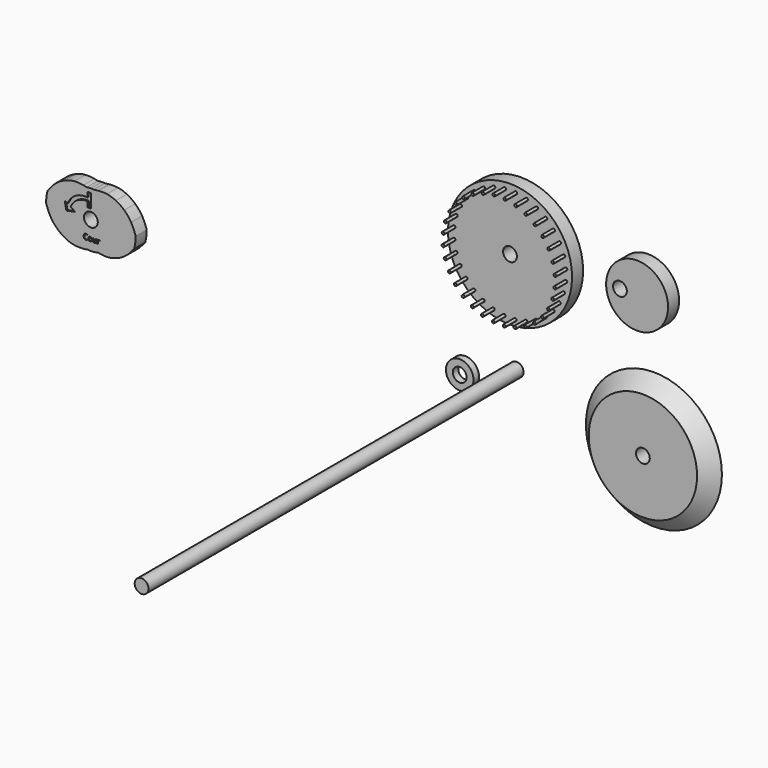
from build123d import *

# Parameters (mm, degrees)
F0_R          = 45
F1_DEPTH      = 10
F0_R_2        = 22.45
F0_R_3        = 49.315
F2_R          = 5
F3_DEPTH      = 10.0010001
F4_R          = 5
F5_DEPTH      = 10.0010001
F6_R          = 5
F7_DEPTH      = 10.0010001
F8_SIZE       = 9.99999
F9_R          = 5
F10_DEPTH     = 340
F11_R         = 10
F12_DEPTH     = 5
F13_R         = 5
F14_DEPTH     = 5.0010001
F16_DEPTH     = 10
F17_R         = 5
F18_DEPTH     = 25
F19_TEXT_SIZE = 5.3993426263
F20_DEPTH     = 1


# Not quite as in the source:
# - a fillet or chamfer is up to 0.001 mm smaller than in the source, because OpenCascade refuses the exact size
# - Text() gives the source's letters only with a copy of the font that has no kerning and outlines rounded to 1/6400 em; it was checked with that copy


with BuildPart() as f1:
    # F0 (on Front) → F1 (new body)
    with BuildSketch(Plane.XZ):
        with Locations((-46.6972251093, 45.5633398328)):
            Circle(F0_R)
    extrude(amount=F1_DEPTH)

    # F2 (on face) → F3 (cut, through all)
    with BuildSketch(Plane.XZ.offset(10)):
        with Locations((-46.6972251093, 45.5633398328)):
            Circle(F2_R)
    extrude(amount=-F3_DEPTH, mode=Mode.SUBTRACT)

    # F15 (on face) → F16 (join)
    with BuildSketch(Plane.XZ.offset(10)):
        with BuildLine():
            Line((-20.3267769857, 14.6089610016), (-21.0381806281, 13.9061773524))
            Line((-21.0381806281, 13.9061773524), (-21.8730211374, 13.3556854596))
            ThreePointArc((-21.8730211374, 13.3556854596), (-20.7508137105, 12.948356777), (-20.0381806281, 13.9061773524))
            ThreePointArc((-20.0381806281, 13.9061773524), (-20.1131391041, 14.2860433535), (-20.3267769857, 14.6089610016))
        make_face()
        with BuildLine():
            Line((-21.8730211374, 13.3556854596), (-21.0381806281, 13.9061773524))
            Line((-21.0381806281, 13.9061773524), (-20.3267769857, 14.6089610016))
            ThreePointArc((-20.3267769857, 14.6089610016), (-21.6678504313, 14.6830402353), (-21.8730211374, 13.3556854596))
        make_face()
        with BuildLine():
            ThreePointArc((-41.4559151977, 86.0920184473), (-42.4528675557, 87.0920138032), (-43.4558966214, 86.0981137029))
            Line((-43.4558966214, 86.0981137029), (-42.4559151977, 86.0920184473))
            Line((-42.4559151977, 86.0920184473), (-41.4763372619, 85.8909536123))
            ThreePointArc((-41.4763372619, 85.8909536123), (-41.4610338138, 85.9909687954), (-41.4559151977, 86.0920184473))
        make_face()
        with BuildLine():
            Line((-42.4559151977, 86.0920184473), (-43.4558966214, 86.0981137029))
            ThreePointArc((-43.4558966214, 86.0981137029), (-42.5599964225, 85.0974496469), (-41.4763372619, 85.8909536123))
            Line((-41.4763372619, 85.8909536123), (-42.4559151977, 86.0920184473))
        make_face()
        with BuildLine():
            ThreePointArc((-49.4441637401, 86.1407097685), (-50.5391474585, 87.1361885946), (-51.4261199266, 85.9516012075))
            Line((-51.4261199266, 85.9516012075), (-50.4441637401, 86.1407097685))
            Line((-50.4441637401, 86.1407097685), (-49.4441823163, 86.1346145129))
            ThreePointArc((-49.4441823163, 86.1346145129), (-49.4441683842, 86.1376621265), (-49.4441637401, 86.1407097685))
        make_face()
        with BuildLine():
            Line((-50.4441637401, 86.1407097685), (-51.4261199266, 85.9516012075))
            ThreePointArc((-51.4261199266, 85.9516012075), (-50.3522143259, 85.1449460891), (-49.4441823163, 86.1346145129))
            Line((-49.4441823163, 86.1346145129), (-50.4441637401, 86.1407097685))
        make_face()
        with BuildLine():
            ThreePointArc((-57.3064633458, 84.8191440801), (-58.5728660212, 85.5887274378), (-59.2146144559, 84.2529904775))
            Line((-59.2146144559, 84.2529904775), (-58.2884195323, 84.6300355191))
            Line((-58.2884195323, 84.6300355191), (-57.3064633458, 84.8191440801))
        make_face()
        with BuildLine():
            Line((-58.2884195323, 84.6300355191), (-59.2146144559, 84.2529904775))
            ThreePointArc((-59.2146144559, 84.2529904775), (-58.0963191987, 83.6486602281), (-57.2884195323, 84.6300355191))
            ThreePointArc((-57.2884195323, 84.6300355191), (-57.2929407062, 84.7250192375), (-57.3064633458, 84.8191440801))
            Line((-57.3064633458, 84.8191440801), (-58.2884195323, 84.6300355191))
        make_face()
        with BuildLine():
            ThreePointArc((-64.7610372996, 81.9950951051), (-66.1532446677, 82.5028282286), (-66.5220727325, 81.0675581706))
            Line((-66.5220727325, 81.0675581706), (-65.6872322232, 81.6180500634))
            Line((-65.6872322232, 81.6180500634), (-64.7610372996, 81.9950951051))
        make_face()
        with BuildLine():
            Line((-65.6872322232, 81.6180500634), (-66.5220727325, 81.0675581706))
            ThreePointArc((-66.5220727325, 81.0675581706), (-65.3998653056, 80.660229488), (-64.6872322232, 81.6180500634))
            ThreePointArc((-64.6872322232, 81.6180500634), (-64.7058569322, 81.810150397), (-64.7610372996, 81.9950951051))
            Line((-64.7610372996, 81.9950951051), (-65.6872322232, 81.6180500634))
        make_face()
        with BuildLine():
            ThreePointArc((-71.5214290812, 77.770994206), (-72.9859393937, 77.9973651962), (-73.0676732328, 76.517718664))
            Line((-73.0676732328, 76.517718664), (-72.3562695905, 77.2205023132))
            Line((-72.3562695905, 77.2205023132), (-71.5214290812, 77.770994206))
        make_face()
        with BuildLine():
            Line((-72.3562695905, 77.2205023132), (-73.0676732328, 76.517718664))
            ThreePointArc((-73.0676732328, 76.517718664), (-71.9764035893, 76.2954607892), (-71.3562695905, 77.2205023132))
            ThreePointArc((-71.3562695905, 77.2205023132), (-71.3984490151, 77.5078692309), (-71.5214290812, 77.770994206))
            Line((-71.5214290812, 77.770994206), (-72.3562695905, 77.2205023132))
        make_face()
        with BuildLine():
            ThreePointArc((-77.3278406257, 72.3091712117), (-78.8083735726, 72.2454807583), (-78.5998722005, 70.7783197384))
            Line((-78.5998722005, 70.7783197384), (-78.0392442681, 71.6063875625))
            Line((-78.0392442681, 71.6063875625), (-77.3278406257, 72.3091712117))
        make_face()
        with BuildLine():
            Line((-78.0392442681, 71.6063875625), (-78.5998722005, 70.7783197384))
            ThreePointArc((-78.5998722005, 70.7783197384), (-77.5705375007, 70.7230337454), (-77.0392442681, 71.6063875625))
            ThreePointArc((-77.0392442681, 71.6063875625), (-77.114202744, 71.9862535636), (-77.3278406257, 72.3091712117))
            Line((-77.3278406257, 72.3091712117), (-78.0392442681, 71.6063875625))
        make_face()
        with BuildLine():
            ThreePointArc((-81.9571347938, 65.8195209167), (-83.3967943242, 65.4682166082), (-82.9060703316, 64.0699232756))
            Line((-82.9060703316, 64.0699232756), (-82.5177627262, 64.9914530926))
            Line((-82.5177627262, 64.9914530926), (-81.9571347938, 65.8195209167))
        make_face()
        with BuildLine():
            Line((-82.5177627262, 64.9914530926), (-82.9060703316, 64.0699232756))
            ThreePointArc((-82.9060703316, 64.0699232756), (-81.964729095, 64.1582941626), (-81.5177627262, 64.9914530926))
            ThreePointArc((-81.5177627262, 64.9914530926), (-81.6344089091, 65.46015986), (-81.9571347938, 65.8195209167))
            Line((-81.9571347938, 65.8195209167), (-82.5177627262, 64.9914530926))
        make_face()
        with BuildLine():
            ThreePointArc((-85.2314104067, 58.5514369425), (-86.5748712122, 57.9260192064), (-85.820782847, 56.6503291898))
            Line((-85.820782847, 56.6503291898), (-85.6197180121, 57.6299071255))
            Line((-85.6197180121, 57.6299071255), (-85.2314104067, 58.5514369425))
        make_face()
        with BuildLine():
            Line((-85.6197180121, 57.6299071255), (-85.820782847, 56.6503291898))
            ThreePointArc((-85.820782847, 56.6503291898), (-84.9876835332, 56.8549668585), (-84.6197180121, 57.6299071255))
            ThreePointArc((-84.6197180121, 57.6299071255), (-84.786559082, 58.1829407568), (-85.2314104067, 58.5514369425))
            Line((-85.2314104067, 58.5514369425), (-85.6197180121, 57.6299071255))
        make_face()
        with BuildLine():
            ThreePointArc((-87.0248388888, 50.7842276802), (-88.2204725241, 49.9087309693), (-87.2319989793, 48.8046683207))
            Line((-87.2319989793, 48.8046683207), (-87.2259037237, 49.8046497444))
            Line((-87.2259037237, 49.8046497444), (-87.0248388888, 50.7842276802))
        make_face()
        with BuildLine():
            Line((-87.2259037237, 49.8046497444), (-87.2319989793, 48.8046683207))
            ThreePointArc((-87.2319989793, 48.8046683207), (-86.5209552347, 49.0953912388), (-86.2259037237, 49.8046497444))
            ThreePointArc((-86.2259037237, 49.8046497444), (-86.4509634567, 50.4366842233), (-87.0248388888, 50.7842276802))
            Line((-87.0248388888, 50.7842276802), (-87.2259037237, 49.8046497444))
        make_face()
        with BuildLine():
            ThreePointArc((-87.2684997893, 42.8163826257), (-88.2703587244, 41.7244517877), (-87.085486484, 40.8344450155))
            Line((-87.085486484, 40.8344450155), (-87.274595045, 41.816401202))
            Line((-87.274595045, 41.816401202), (-87.2684997893, 42.8163826257))
        make_face()
        with BuildLine():
            Line((-87.274595045, 41.816401202), (-87.085486484, 40.8344450155))
            ThreePointArc((-87.085486484, 40.8344450155), (-86.5035215851, 41.1796550049), (-86.274595045, 41.816401202))
            ThreePointArc((-86.274595045, 41.816401202), (-86.5653365393, 42.521349691), (-87.2684997893, 42.8163826257))
            Line((-87.2684997893, 42.8163826257), (-87.274595045, 41.816401202))
        make_face()
        with BuildLine():
            ThreePointArc((-85.9530293566, 34.9541015963), (-86.7226127143, 33.6876989209), (-85.386875754, 33.0459504862))
            Line((-85.386875754, 33.0459504862), (-85.7639207956, 33.9721454098))
            Line((-85.7639207956, 33.9721454098), (-85.9530293566, 34.9541015963))
        make_face()
        with BuildLine():
            Line((-85.7639207956, 33.9721454098), (-85.386875754, 33.0459504862))
            ThreePointArc((-85.386875754, 33.0459504862), (-84.9341482239, 33.4140437352), (-84.7639207956, 33.9721454098))
            ThreePointArc((-84.7639207956, 33.9721454098), (-85.1271745985, 34.7432188697), (-85.9530293566, 34.9541015963))
            Line((-85.9530293566, 34.9541015963), (-85.7639207956, 33.9721454098))
        make_face()
        with BuildLine():
            ThreePointArc((-83.1289803815, 27.4995276425), (-83.6367135051, 26.1073202744), (-82.2014434471, 25.7384922096))
            Line((-82.2014434471, 25.7384922096), (-82.7519353399, 26.5733327189))
            Line((-82.7519353399, 26.5733327189), (-83.1289803815, 27.4995276425))
        make_face()
        with BuildLine():
            Line((-82.7519353399, 26.5733327189), (-82.2014434471, 25.7384922096))
            ThreePointArc((-82.2014434471, 25.7384922096), (-81.8714548197, 26.099250391), (-81.7519353399, 26.5733327189))
            ThreePointArc((-81.7519353399, 26.5733327189), (-82.1938336653, 27.4031052906), (-83.1289803815, 27.4995276425))
            Line((-83.1289803815, 27.4995276425), (-82.7519353399, 26.5733327189))
        make_face()
        with BuildLine():
            ThreePointArc((-78.9048794825, 20.7391358609), (-79.1312504727, 19.2746255484), (-77.6516039405, 19.1928917093))
            Line((-77.6516039405, 19.1928917093), (-78.3543875897, 19.9042953516))
            Line((-78.3543875897, 19.9042953516), (-78.9048794825, 20.7391358609))
        make_face()
        with BuildLine():
            Line((-78.3543875897, 19.9042953516), (-77.6516039405, 19.1928917093))
            ThreePointArc((-77.6516039405, 19.1928917093), (-77.4316786299, 19.5187980424), (-77.3543875897, 19.9042953516))
            ThreePointArc((-77.3543875897, 19.9042953516), (-77.8803052618, 20.7847758718), (-78.9048794825, 20.7391358609))
            Line((-78.9048794825, 20.7391358609), (-78.3543875897, 19.9042953516))
        make_face()
        with BuildLine():
            ThreePointArc((-73.4430564882, 14.9327243164), (-73.3793660348, 13.4521913695), (-71.9122050148, 13.6606927416))
            Line((-71.9122050148, 13.6606927416), (-72.740272839, 14.221320674))
            Line((-72.740272839, 14.221320674), (-73.4430564882, 14.9327243164))
        make_face()
        with BuildLine():
            Line((-72.740272839, 14.221320674), (-71.9122050148, 13.6606927416))
            ThreePointArc((-71.9122050148, 13.6606927416), (-71.7842216311, 13.9281209334), (-71.740272839, 14.221320674))
            ThreePointArc((-71.740272839, 14.221320674), (-72.3547755298, 15.1440296339), (-73.4430564882, 14.9327243164))
            Line((-73.4430564882, 14.9327243164), (-72.740272839, 14.221320674))
        make_face()
        with BuildLine():
            ThreePointArc((-66.9534061932, 10.3034301483), (-66.6021018846, 8.8637706179), (-65.2038085521, 9.3544946105))
            Line((-65.2038085521, 9.3544946105), (-66.1253383691, 9.7428022159))
            Line((-66.1253383691, 9.7428022159), (-66.9534061932, 10.3034301483))
        make_face()
        with BuildLine():
            Line((-66.1253383691, 9.7428022159), (-65.2038085521, 9.3544946105))
            ThreePointArc((-65.2038085521, 9.3544946105), (-65.145152209, 9.5447237175), (-65.1253383691, 9.7428022159))
            ThreePointArc((-65.1253383691, 9.7428022159), (-65.8321386284, 10.6988534238), (-66.9534061932, 10.3034301483))
            Line((-66.9534061932, 10.3034301483), (-66.1253383691, 9.7428022159))
        make_face()
        with BuildLine():
            ThreePointArc((-59.685322219, 7.0291545354), (-59.0599044828, 5.6856937299), (-57.7842144663, 6.439782095))
            Line((-57.7842144663, 6.439782095), (-58.763792402, 6.64084693))
            Line((-58.763792402, 6.64084693), (-59.685322219, 7.0291545354))
        make_face()
        with BuildLine():
            Line((-58.763792402, 6.64084693), (-57.7842144663, 6.439782095))
            ThreePointArc((-57.7842144663, 6.439782095), (-57.7689110182, 6.5397972781), (-57.763792402, 6.64084693))
            ThreePointArc((-57.763792402, 6.64084693), (-58.5657139036, 7.6210330901), (-59.685322219, 7.0291545354))
            Line((-59.685322219, 7.0291545354), (-58.763792402, 6.64084693))
        make_face()
        with BuildLine():
            ThreePointArc((-51.9181129566, 5.2357260533), (-51.0426162457, 4.040092418), (-49.9385535972, 5.0285659628))
            Line((-49.9385535972, 5.0285659628), (-50.9385350209, 5.0346612184))
            Line((-50.9385350209, 5.0346612184), (-51.9181129566, 5.2357260533))
        make_face()
        with BuildLine():
            Line((-50.9385350209, 5.0346612184), (-49.9385535972, 5.0285659628))
            ThreePointArc((-49.9385535972, 5.0285659628), (-49.938539665, 5.0316135764), (-49.9385350209, 5.0346612184))
            ThreePointArc((-49.9385350209, 5.0346612184), (-50.8374853691, 6.0295426022), (-51.9181129566, 5.2357260533))
            Line((-51.9181129566, 5.2357260533), (-50.9385350209, 5.0346612184))
        make_face()
        with BuildLine():
            ThreePointArc((-41.9502864785, 4.9859698971), (-41.9548076523, 5.0809536155), (-41.968330292, 5.1750784581))
            Line((-41.968330292, 5.1750784581), (-42.9502864785, 4.9859698971))
            Line((-42.9502864785, 4.9859698971), (-43.9502679022, 4.9920651527))
            ThreePointArc((-43.9502679022, 4.9920651527), (-42.9533341204, 3.9859745412), (-41.9502864785, 4.9859698971))
        make_face()
        with BuildLine():
            Line((-42.9502864785, 4.9859698971), (-41.968330292, 5.1750784581))
            ThreePointArc((-41.968330292, 5.1750784581), (-43.0422358927, 5.9817335765), (-43.9502679022, 4.9920651527))
            Line((-43.9502679022, 4.9920651527), (-42.9502864785, 4.9859698971))
        make_face()
        with BuildLine():
            ThreePointArc((-34.1060306863, 6.4966441465), (-34.1246553953, 6.6887444801), (-34.1798357626, 6.8736891881))
            Line((-34.1798357626, 6.8736891881), (-35.1060306863, 6.4966441465))
            Line((-35.1060306863, 6.4966441465), (-36.0879868727, 6.3075355855))
            ThreePointArc((-36.0879868727, 6.3075355855), (-35.0110469679, 5.5011653204), (-34.1060306863, 6.4966441465))
        make_face()
        with BuildLine():
            Line((-35.1060306863, 6.4966441465), (-34.1798357626, 6.8736891881))
            ThreePointArc((-34.1798357626, 6.8736891881), (-35.3904771752, 7.4553360652), (-36.0879868727, 6.3075355855))
            Line((-36.0879868727, 6.3075355855), (-35.1060306863, 6.4966441465))
        make_face()
        with BuildLine():
            ThreePointArc((-26.7072179953, 9.5086296022), (-26.74939742, 9.7959965198), (-26.8723774861, 10.059121495))
            Line((-26.8723774861, 10.059121495), (-27.7072179953, 9.5086296022))
            Line((-27.7072179953, 9.5086296022), (-28.633412919, 9.1315845606))
            ThreePointArc((-28.633412919, 9.1315845606), (-27.5151176617, 8.5272543112), (-26.7072179953, 9.5086296022))
        make_face()
        with BuildLine():
            Line((-27.7072179953, 9.5086296022), (-26.8723774861, 10.059121495))
            ThreePointArc((-26.8723774861, 10.059121495), (-28.1732304399, 10.3934077674), (-28.633412919, 9.1315845606))
            Line((-28.633412919, 9.1315845606), (-27.7072179953, 9.5086296022))
        make_face()
        with BuildLine():
            ThreePointArc((-35.6102357523, 84.6868975706), (-34.9267698973, 83.5306795356), (-33.7091279996, 84.0975251302))
            Line((-33.7091279996, 84.0975251302), (-34.6306578165, 84.4858327356))
            Line((-34.6306578165, 84.4858327356), (-35.6102357523, 84.6868975706))
        make_face()
        with BuildLine():
            Line((-34.6306578165, 84.4858327356), (-33.7091279996, 84.0975251302))
            ThreePointArc((-33.7091279996, 84.0975251302), (-33.6504716564, 84.2877542373), (-33.6306578165, 84.4858327356))
            ThreePointArc((-33.6306578165, 84.4858327356), (-34.5296081647, 85.4807141194), (-35.6102357523, 84.6868975706))
            Line((-35.6102357523, 84.6868975706), (-34.6306578165, 84.4858327356))
        make_face()
        with BuildLine():
            ThreePointArc((-28.1906416665, 81.7721850552), (-27.7458753651, 80.5048458518), (-26.4410440253, 80.8232495173))
            Line((-26.4410440253, 80.8232495173), (-27.2691118495, 81.3838774497))
            Line((-27.2691118495, 81.3838774497), (-28.1906416665, 81.7721850552))
        make_face()
        with BuildLine():
            Line((-27.2691118495, 81.3838774497), (-26.4410440253, 80.8232495173))
            ThreePointArc((-26.4410440253, 80.8232495173), (-26.3130606416, 81.0906777091), (-26.2691118495, 81.3838774497))
            ThreePointArc((-26.2691118495, 81.3838774497), (-27.0710333511, 82.3640636098), (-28.1906416665, 81.7721850552))
            Line((-28.1906416665, 81.7721850552), (-27.2691118495, 81.3838774497))
        make_face()
        with BuildLine():
            ThreePointArc((-21.4822452037, 77.465986924), (-21.2932705754, 76.1362296871), (-19.9513937304, 76.1939553492))
            Line((-19.9513937304, 76.1939553492), (-20.6541773796, 76.9053589916))
            Line((-20.6541773796, 76.9053589916), (-21.4822452037, 77.465986924))
        make_face()
        with BuildLine():
            Line((-20.6541773796, 76.9053589916), (-19.9513937304, 76.1939553492))
            ThreePointArc((-19.9513937304, 76.1939553492), (-19.7314684197, 76.5198616824), (-19.6541773796, 76.9053589916))
            ThreePointArc((-19.6541773796, 76.9053589916), (-20.3609776389, 77.8614101995), (-21.4822452037, 77.465986924))
            Line((-21.4822452037, 77.465986924), (-20.6541773796, 76.9053589916))
        make_face()
        with BuildLine():
            ThreePointArc((-15.7428462781, 71.9337879564), (-15.8169255118, 70.5927145108), (-14.489570736, 70.3875438047))
            Line((-14.489570736, 70.3875438047), (-15.0400626288, 71.222384314))
            Line((-15.0400626288, 71.222384314), (-15.7428462781, 71.9337879564))
        make_face()
        with BuildLine():
            Line((-15.0400626288, 71.222384314), (-14.489570736, 70.3875438047))
            ThreePointArc((-14.489570736, 70.3875438047), (-14.1595821087, 70.7483019861), (-14.0400626288, 71.222384314))
            ThreePointArc((-14.0400626288, 71.222384314), (-14.6545653197, 72.1450932739), (-15.7428462781, 71.9337879564))
            Line((-15.7428462781, 71.9337879564), (-15.0400626288, 71.222384314))
        make_face()
        with BuildLine():
            ThreePointArc((-11.1930067715, 65.388187456), (-11.5272930438, 64.0873345022), (-10.265469837, 63.6271520231))
            Line((-10.265469837, 63.6271520231), (-10.6425148787, 64.5533469467))
            Line((-10.6425148787, 64.5533469467), (-11.1930067715, 65.388187456))
        make_face()
        with BuildLine():
            Line((-10.6425148787, 64.5533469467), (-10.265469837, 63.6271520231))
            ThreePointArc((-10.265469837, 63.6271520231), (-9.8127423069, 63.9952452722), (-9.6425148787, 64.5533469467))
            ThreePointArc((-9.6425148787, 64.5533469467), (-10.1684325508, 65.4338274669), (-11.1930067715, 65.388187456))
            Line((-11.1930067715, 65.388187456), (-10.6425148787, 64.5533469467))
        make_face()
        with BuildLine():
            ThreePointArc((-8.0075744646, 58.0807291795), (-8.5892213416, 56.8700877669), (-7.441420862, 56.1725780693))
            Line((-7.441420862, 56.1725780693), (-7.630529423, 57.1545342558))
            Line((-7.630529423, 57.1545342558), (-8.0075744646, 58.0807291795))
        make_face()
        with BuildLine():
            Line((-7.630529423, 57.1545342558), (-7.441420862, 56.1725780693))
            ThreePointArc((-7.441420862, 56.1725780693), (-6.8594559631, 56.5177880587), (-6.630529423, 57.1545342558))
            ThreePointArc((-6.630529423, 57.1545342558), (-7.0724277484, 57.9843068276), (-8.0075744646, 58.0807291795))
            Line((-8.0075744646, 58.0807291795), (-7.630529423, 57.1545342558))
        make_face()
        with BuildLine():
            ThreePointArc((-6.3089637346, 50.2922346501), (-7.115618853, 49.2183290494), (-6.1259504292, 48.3102970399))
            Line((-6.1259504292, 48.3102970399), (-6.1198551736, 49.3102784636))
            Line((-6.1198551736, 49.3102784636), (-6.3089637346, 50.2922346501))
        make_face()
        with BuildLine():
            Line((-6.1198551736, 49.3102784636), (-6.1259504292, 48.3102970399))
            ThreePointArc((-6.1259504292, 48.3102970399), (-5.4149066846, 48.601019958), (-5.1198551736, 49.3102784636))
            ThreePointArc((-5.1198551736, 49.3102784636), (-5.4831089765, 50.0813519235), (-6.3089637346, 50.2922346501))
            Line((-6.3089637346, 50.2922346501), (-6.1198551736, 49.3102784636))
        make_face()
        with BuildLine():
            ThreePointArc((-6.1624512392, 42.3220113449), (-7.1631152952, 41.426111146), (-6.3696113298, 40.3424519855))
            Line((-6.3696113298, 40.3424519855), (-6.1685464948, 41.3220299212))
            Line((-6.1685464948, 41.3220299212), (-6.1624512392, 42.3220113449))
        make_face()
        with BuildLine():
            Line((-6.1685464948, 41.3220299212), (-6.3696113298, 40.3424519855))
            ThreePointArc((-6.3696113298, 40.3424519855), (-5.5365120159, 40.5470896541), (-5.1685464948, 41.3220299212))
            ThreePointArc((-5.1685464948, 41.3220299212), (-5.4592879892, 42.0269784102), (-6.1624512392, 42.3220113449))
            Line((-6.1624512392, 42.3220113449), (-6.1685464948, 41.3220299212))
        make_face()
        with BuildLine():
            ThreePointArc((-7.5736673715, 34.4763504758), (-8.7298854065, 33.7928846209), (-8.1630398119, 32.5752427231))
            Line((-8.1630398119, 32.5752427231), (-7.7747322065, 33.4967725401))
            Line((-7.7747322065, 33.4967725401), (-7.5736673715, 34.4763504758))
        make_face()
        with BuildLine():
            Line((-7.7747322065, 33.4967725401), (-8.1630398119, 32.5752427231))
            ThreePointArc((-8.1630398119, 32.5752427231), (-7.2216985752, 32.66361361), (-6.7747322065, 33.4967725401))
            ThreePointArc((-6.7747322065, 33.4967725401), (-6.9997919394, 34.128807019), (-7.5736673715, 34.4763504758))
            Line((-7.5736673715, 34.4763504758), (-7.7747322065, 33.4967725401))
        make_face()
        with BuildLine():
            ThreePointArc((-10.4883798869, 27.05675639), (-11.7557190903, 26.6119900886), (-11.4373154248, 25.3071587489))
            Line((-11.4373154248, 25.3071587489), (-10.8766874924, 26.135226573))
            Line((-10.8766874924, 26.135226573), (-10.4883798869, 27.05675639))
        make_face()
        with BuildLine():
            Line((-10.8766874924, 26.135226573), (-11.4373154248, 25.3071587489))
            ThreePointArc((-11.4373154248, 25.3071587489), (-10.407980725, 25.2518727559), (-9.8766874924, 26.135226573))
            ThreePointArc((-9.8766874924, 26.135226573), (-10.0435285623, 26.6882602043), (-10.4883798869, 27.05675639))
            Line((-10.4883798869, 27.05675639), (-10.8766874924, 26.135226573))
        make_face()
        with BuildLine():
            ThreePointArc((-14.7945780181, 20.3483599273), (-16.124335255, 20.1593852989), (-16.0666095929, 18.8175084539))
            Line((-16.0666095929, 18.8175084539), (-15.3552059505, 19.5202921031))
            Line((-15.3552059505, 19.5202921031), (-14.7945780181, 20.3483599273))
        make_face()
        with BuildLine():
            Line((-15.3552059505, 19.5202921031), (-16.0666095929, 18.8175084539))
            ThreePointArc((-16.0666095929, 18.8175084539), (-14.9753399494, 18.5952505791), (-14.3552059505, 19.5202921031))
            ThreePointArc((-14.3552059505, 19.5202921031), (-14.4718521334, 19.9889988705), (-14.7945780181, 20.3483599273))
            Line((-14.7945780181, 20.3483599273), (-15.3552059505, 19.5202921031))
        make_face()
    extrude(amount=F16_DEPTH)


with BuildPart() as f1b:
    # F0 (on Front) → F1, piece 2 (new body)
    with BuildSketch(Plane.XZ):
        with Locations((45.457674756, 49.0673256573)):
            Circle(F0_R_2)
    extrude(amount=F1_DEPTH)

    # F6 (on face) → F7 (cut, through all)
    with BuildSketch(Plane.XZ.offset(10)):
        with Locations((33.0115074419, 49.3762256208)):
            Circle(F6_R)
    extrude(amount=-F7_DEPTH, mode=Mode.SUBTRACT)


with BuildPart() as f1c:
    # F0 (on Front) → F1, piece 3 (new body)
    with BuildSketch(Plane.XZ):
        with Locations((49.6624586107, -51.8475387692)):
            Circle(F0_R_3)
    extrude(amount=F1_DEPTH)

    # F4 (on face) → F5 (cut, through all)
    with BuildSketch(Plane.XZ.offset(10)):
        with Locations((49.6624586107, -51.8475387692)):
            Circle(F4_R)
    extrude(amount=-F5_DEPTH, mode=Mode.SUBTRACT)

    # F8 (size 10 in the source; OpenCascade refuses exactly that, so slightly less here)
    f8_edges = [f1c.edges().sort_by_distance(p)[0] for p in [
        (0.347459, -10, -51.847539),
    ]]
    chamfer(f8_edges, length=F8_SIZE)


with BuildPart() as f1d:
    # F0 (on Front) → F1, piece 4 (new body)
    with BuildSketch(Plane.XZ):
        with BuildLine():
            ThreePointArc((-331.3206634485, -36.470353457), (-330.8102827468, -33.9044963994), (-330.6391799743, -31.293972555))
            ThreePointArc((-330.6391799743, -31.293972555), (-330.8102827468, -28.6834487106), (-331.3206634485, -26.1175916529))
            ThreePointArc((-331.3206634485, -26.1175916529), (-332.1615893241, -23.6403039077), (-333.3186718986, -21.293972555))
            ThreePointArc((-333.3186718986, -21.293972555), (-334.7721131685, -19.1187439748), (-336.4970443506, -17.1518369312))
            ThreePointArc((-336.4970443506, -17.1518369312), (-338.4639513941, -15.4269057491), (-340.6391799743, -13.9734644793))
            ThreePointArc((-340.6391799743, -13.9734644793), (-342.985511327, -12.8163819047), (-345.4627990723, -11.9754560292))
            ThreePointArc((-345.4627990723, -11.9754560292), (-347.037380693, -11.6209696846), (-348.6354187421, -11.3946021899))
            ThreePointArc((-348.6354187421, -11.3946021899), (-349.6360367394, -11.319145806), (-350.6391799743, -11.293972555))
            ThreePointArc((-350.6391799743, -11.293972555), (-352.1457160849, -11.3507945497), (-353.6436917567, -11.5209376602))
            ThreePointArc((-353.6436917567, -11.5209376602), (-354.7359345454, -11.7180536242), (-355.8155608764, -11.9754560292))
            ThreePointArc((-355.8155608764, -11.9754560292), (-358.2928486216, -12.8163819047), (-360.6391799743, -13.9734644793))
            ThreePointArc((-360.6391799743, -13.9734644793), (-362.8144085545, -15.4269057491), (-364.781315598, -17.1518369312))
            ThreePointArc((-364.781315598, -17.1518369312), (-366.5062467801, -19.1187439748), (-367.95968805, -21.293972555))
            ThreePointArc((-367.95968805, -21.293972555), (-369.1167706245, -23.6403039077), (-369.9576965001, -26.1175916529))
            ThreePointArc((-369.9576965001, -26.1175916529), (-370.4680772018, -28.6834487106), (-370.6391799743, -31.293972555))
            ThreePointArc((-370.6391799743, -31.293972555), (-370.4680772018, -33.9044963994), (-369.9576965001, -36.470353457))
            ThreePointArc((-369.9576965001, -36.470353457), (-369.1167706245, -38.9476412023), (-367.95968805, -41.293972555))
            ThreePointArc((-367.95968805, -41.293972555), (-366.5062467801, -43.4692011351), (-364.781315598, -45.4361081787))
            ThreePointArc((-364.781315598, -45.4361081787), (-362.8144085545, -47.1610393608), (-360.6391799743, -48.6144806306))
            ThreePointArc((-360.6391799743, -48.6144806306), (-358.2928486216, -49.7715632052), (-355.8155608764, -50.6124890807))
            ThreePointArc((-355.8155608764, -50.6124890807), (-354.2394341305, -50.9672582493), (-352.6398153961, -51.1936574246))
            ThreePointArc((-352.6398153961, -51.1936574246), (-351.6407543869, -51.268878029), (-350.6391799743, -51.293972555))
            ThreePointArc((-350.6391799743, -51.293972555), (-348.0286561299, -51.1228697824), (-345.4627990723, -50.6124890807))
            ThreePointArc((-345.4627990723, -50.6124890807), (-342.985511327, -49.7715632052), (-340.6391799743, -48.6144806306))
            ThreePointArc((-340.6391799743, -48.6144806306), (-338.4639513941, -47.1610393608), (-336.4970443506, -45.4361081787))
            ThreePointArc((-336.4970443506, -45.4361081787), (-334.7721131685, -43.4692011351), (-333.3186718986, -41.293972555))
            ThreePointArc((-333.3186718986, -41.293972555), (-332.1615893241, -38.9476412023), (-331.3206634485, -36.470353457))
        make_face()
        with BuildLine():
            Line((-318.1391799743, -31.293972555), (-330.6391799743, -31.293972555))
            ThreePointArc((-330.6391799743, -31.293972555), (-330.8102827468, -33.9044963994), (-331.3206634485, -36.470353457))
            Line((-331.3206634485, -36.470353457), (-319.2465906199, -39.7055915208))
            ThreePointArc((-319.2465906199, -39.7055915208), (-318.4172219797, -35.5360738021), (-318.1391799743, -31.293972555))
        make_face()
        with BuildLine():
            ThreePointArc((-331.3206634485, -26.1175916529), (-330.8102827468, -28.6834487106), (-330.6391799743, -31.293972555))
            Line((-330.6391799743, -31.293972555), (-318.1391799743, -31.293972555))
            add(Edge.make_bspline(
                [(-321.4682200204, -23.4776373929), (-320.0791480854, -25.8891723509), (-319.1091640299, -28.5915724529), (-318.1391799743, -31.293972555)],
                knots=[0.8106564665, 0.8106564665, 0.8106564665, 0.8106564665, 1, 1, 1, 1], degree=3))
            Line((-321.4682200204, -23.4776373929), (-331.3206634485, -26.1175916529))
        make_face()
        with BuildLine():
            ThreePointArc((-333.3186718986, -21.293972555), (-332.1615893241, -23.6403039077), (-331.3206634485, -26.1175916529))
            Line((-331.3206634485, -26.1175916529), (-321.4682200204, -23.4776373929))
            add(Edge.make_bspline(
                [(-326.4770712087, -17.343972555), (-324.5410444938, -19.0922749893), (-322.8093135762, -21.149396565), (-321.4682200204, -23.4776373929)],
                knots=[0.627852836, 0.627852836, 0.627852836, 0.627852836, 0.8106564665, 0.8106564665, 0.8106564665, 0.8106564665], degree=3))
            Line((-326.4770712087, -17.343972555), (-333.3186718986, -21.293972555))
        make_face()
        with BuildLine():
            Line((-319.2465906199, -39.7055915208), (-331.3206634485, -36.470353457))
            ThreePointArc((-331.3206634485, -36.470353457), (-332.1615893241, -38.9476412023), (-333.3186718986, -41.293972555))
            Line((-333.3186718986, -41.293972555), (-325.2040138652, -45.978972555))
            add(Edge.make_bspline(
                [(-319.2465906199, -39.7055915208), (-321.1336024153, -41.9533240414), (-323.0206142106, -44.201056562), (-325.2040138652, -45.978972555)],
                knots=[0, 0, 0, 0, 0.2683906872, 0.2683906872, 0.2683906872, 0.2683906872], degree=3))
        make_face()
        with BuildLine():
            ThreePointArc((-336.4970443506, -17.1518369312), (-334.7721131685, -19.1187439748), (-333.3186718986, -21.293972555))
            Line((-333.3186718986, -21.293972555), (-326.4770712087, -17.343972555))
            add(Edge.make_bspline(
                [(-332.5372463759, -13.1920389566), (-330.395934388, -14.2627108581), (-328.3417454917, -15.6601039579), (-326.4770712087, -17.343972555)],
                knots=[0.4517864492, 0.4517864492, 0.4517864492, 0.4517864492, 0.627852836, 0.627852836, 0.627852836, 0.627852836], degree=3))
            Line((-332.5372463759, -13.1920389566), (-336.4970443506, -17.1518369312))
        make_face()
        with BuildLine():
            Line((-325.2040138652, -45.978972555), (-333.3186718986, -41.293972555))
            ThreePointArc((-333.3186718986, -41.293972555), (-334.7721131685, -43.4692011351), (-336.4970443506, -45.4361081787))
            Line((-336.4970443506, -45.4361081787), (-332.0776269682, -49.8555255611))
            add(Edge.make_bspline(
                [(-325.2040138652, -45.978972555), (-327.2893106377, -47.6770045548), (-329.6449594667, -48.9464904436), (-332.0776269682, -49.8555255611)],
                knots=[0.2683906872, 0.2683906872, 0.2683906872, 0.2683906872, 0.5247222446, 0.5247222446, 0.5247222446, 0.5247222446], degree=3))
        make_face()
        with BuildLine():
            ThreePointArc((-340.6391799743, -13.9734644793), (-338.4639513941, -15.4269057491), (-336.4970443506, -17.1518369312))
            Line((-336.4970443506, -17.1518369312), (-332.5372463759, -13.1920389566))
            add(Edge.make_bspline(
                [(-338.9891799743, -11.1155806468), (-336.7312968284, -11.436625491), (-334.5940794305, -12.1636071493), (-332.5372463759, -13.1920389566)],
                knots=[0.2826662246, 0.2826662246, 0.2826662246, 0.2826662246, 0.4517864492, 0.4517864492, 0.4517864492, 0.4517864492], degree=3))
            Line((-338.9891799743, -11.1155806468), (-340.6391799743, -13.9734644793))
        make_face()
        with BuildLine():
            Line((-332.0776269682, -49.8555255611), (-336.4970443506, -45.4361081787))
            ThreePointArc((-336.4970443506, -45.4361081787), (-338.4639513941, -47.1610393608), (-340.6391799743, -48.6144806306))
            Line((-340.6391799743, -48.6144806306), (-339.0791799743, -51.3164798905))
            add(Edge.make_bspline(
                [(-332.0776269682, -49.8555255611), (-334.3935818988, -50.7209477206), (-336.7793425041, -51.2596762552), (-339.0791799743, -51.3164798905)],
                knots=[0.5247222446, 0.5247222446, 0.5247222446, 0.5247222446, 0.768755732, 0.768755732, 0.768755732, 0.768755732], degree=3))
        make_face()
        with BuildLine():
            ThreePointArc((-345.4627990723, -11.9754560292), (-342.985511327, -12.8163819047), (-340.6391799743, -13.9734644793))
            Line((-340.6391799743, -13.9734644793), (-338.9891799743, -11.1155806468))
            add(Edge.make_bspline(
                [(-345.2039800272, -11.0095302029), (-343.4242888791, -10.8729632986), (-341.1514054001, -10.808137223), (-338.9891799743, -11.1155806468)],
                knots=[0.1207109657, 0.1207109657, 0.1207109657, 0.1207109657, 0.2826662246, 0.2826662246, 0.2826662246, 0.2826662246], degree=3))
            Line((-345.2039800272, -11.0095302029), (-345.4627990723, -11.9754560292))
        make_face()
        with BuildLine():
            Line((-339.0791799743, -51.3164798905), (-340.6391799743, -48.6144806306))
            ThreePointArc((-340.6391799743, -48.6144806306), (-342.985511327, -49.7715632052), (-345.4627990723, -50.6124890807))
            add(Edge.make_bspline(
                [(-339.0791799743, -51.3164798905), (-341.2584883873, -51.3703065812), (-343.3606437298, -50.991397831), (-345.4627990723, -50.6124890807)],
                knots=[0.768755732, 0.768755732, 0.768755732, 0.768755732, 1, 1, 1, 1], degree=3))
        make_face()
        with BuildLine():
            ThreePointArc((-348.6354187421, -11.3946021899), (-347.037380693, -11.6209696846), (-345.4627990723, -11.9754560292))
            Line((-345.4627990723, -11.9754560292), (-345.2039800272, -11.0095302029))
            add(Edge.make_bspline(
                [(-348.6354187421, -11.3946021899), (-347.5829326704, -11.2529602612), (-346.5304465987, -11.1113183325), (-345.2039800272, -11.0095302029)],
                knots=[0, 0, 0, 0, 0.1207109657, 0.1207109657, 0.1207109657, 0.1207109657], degree=3))
        make_face()
        with BuildLine():
            add(Edge.make_bspline(
                [(-352.6398153961, -51.1936574246), (-353.6934040957, -51.3351662186), (-354.7469927953, -51.4766750126), (-356.0743799215, -51.578414907)],
                knots=[0, 0, 0, 0, 0.1207581565, 0.1207581565, 0.1207581565, 0.1207581565], degree=3))
            ThreePointArc((-352.6398153961, -51.1936574246), (-354.2394341305, -50.9672582493), (-355.8155608764, -50.6124890807))
            Line((-355.8155608764, -50.6124890807), (-356.0743799215, -51.578414907))
        make_face()
        with BuildLine():
            ThreePointArc((-355.8155608764, -11.9754560292), (-354.7359345454, -11.7180536242), (-353.6436917567, -11.5209376602))
            add(Edge.make_bspline(
                [(-356.0743799215, -11.0095302029), (-355.0493997027, -11.1789532798), (-354.3465457297, -11.34994547), (-353.6436917567, -11.5209376602)],
                knots=[0.8744321336, 0.8744321336, 0.8744321336, 0.8744321336, 1, 1, 1, 1], degree=3))
            Line((-356.0743799215, -11.0095302029), (-355.8155608764, -11.9754560292))
        make_face()
        with BuildLine():
            Line((-356.0743799215, -51.578414907), (-355.8155608764, -50.6124890807))
            ThreePointArc((-355.8155608764, -50.6124890807), (-358.2928486216, -49.7715632052), (-360.6391799743, -48.6144806306))
            Line((-360.6391799743, -48.6144806306), (-362.2891799743, -51.4723644631))
            add(Edge.make_bspline(
                [(-356.0743799215, -51.578414907), (-357.8545146496, -51.7148564287), (-360.1270759624, -51.779773568), (-362.2891799743, -51.4723644631)],
                knots=[0.1207581565, 0.1207581565, 0.1207581565, 0.1207581565, 0.2827047234, 0.2827047234, 0.2827047234, 0.2827047234], degree=3))
        make_face()
        with BuildLine():
            ThreePointArc((-360.6391799743, -13.9734644793), (-358.2928486216, -12.8163819047), (-355.8155608764, -11.9754560292))
            Line((-355.8155608764, -11.9754560292), (-356.0743799215, -11.0095302029))
            add(Edge.make_bspline(
                [(-362.5741799743, -10.6219461666), (-360.2378534811, -10.4650249719), (-357.7339033751, -10.7352209386), (-356.0743799215, -11.0095302029)],
                knots=[0.6711278985, 0.6711278985, 0.6711278985, 0.6711278985, 0.8744321336, 0.8744321336, 0.8744321336, 0.8744321336], degree=3))
            Line((-362.5741799743, -10.6219461666), (-360.6391799743, -13.9734644793))
        make_face()
        with BuildLine():
            Line((-362.2891799743, -51.4723644631), (-360.6391799743, -48.6144806306))
            ThreePointArc((-360.6391799743, -48.6144806306), (-362.8144085545, -47.1610393608), (-364.781315598, -45.4361081787))
            Line((-364.781315598, -45.4361081787), (-368.7411135727, -49.3959061533))
            add(Edge.make_bspline(
                [(-362.2891799743, -51.4723644631), (-364.546936335, -51.1513554561), (-366.6842458557, -50.4243477583), (-368.7411135727, -49.3959061533)],
                knots=[0.2827047234, 0.2827047234, 0.2827047234, 0.2827047234, 0.4518158714, 0.4518158714, 0.4518158714, 0.4518158714], degree=3))
        make_face()
        with BuildLine():
            ThreePointArc((-364.781315598, -17.1518369312), (-362.8144085545, -15.4269057491), (-360.6391799743, -13.9734644793))
            Line((-360.6391799743, -13.9734644793), (-362.5741799743, -10.6219461666))
            add(Edge.make_bspline(
                [(-369.5542863711, -12.3788661582), (-367.3016801571, -11.4240651537), (-365.0305779705, -10.7869320577), (-362.5741799743, -10.6219461666)],
                knots=[0.4573751901, 0.4573751901, 0.4573751901, 0.4573751901, 0.6711278985, 0.6711278985, 0.6711278985, 0.6711278985], degree=3))
            Line((-369.5542863711, -12.3788661582), (-364.781315598, -17.1518369312))
        make_face()
        with BuildLine():
            Line((-368.7411135727, -49.3959061533), (-364.781315598, -45.4361081787))
            ThreePointArc((-364.781315598, -45.4361081787), (-366.5062467801, -43.4692011351), (-367.95968805, -41.293972555))
            Line((-367.95968805, -41.293972555), (-374.8012887399, -45.243972555))
            add(Edge.make_bspline(
                [(-368.7411135727, -49.3959061533), (-370.8824616467, -48.3252240517), (-372.9366243517, -46.9278383551), (-374.8012887399, -45.243972555)],
                knots=[0.4518158714, 0.4518158714, 0.4518158714, 0.4518158714, 0.6278728089, 0.6278728089, 0.6278728089, 0.6278728089], degree=3))
        make_face()
        with BuildLine():
            ThreePointArc((-367.95968805, -21.293972555), (-366.5062467801, -19.1187439748), (-364.781315598, -17.1518369312))
            Line((-364.781315598, -17.1518369312), (-369.5542863711, -12.3788661582))
            add(Edge.make_bspline(
                [(-376.2908524344, -16.483972555), (-374.250519467, -14.7261911279), (-371.9125386988, -13.3784468561), (-369.5542863711, -12.3788661582)],
                knots=[0.2335975858, 0.2335975858, 0.2335975858, 0.2335975858, 0.4573751901, 0.4573751901, 0.4573751901, 0.4573751901], degree=3))
            Line((-376.2908524344, -16.483972555), (-367.95968805, -21.293972555))
        make_face()
        with BuildLine():
            Line((-374.8012887399, -45.243972555), (-367.95968805, -41.293972555))
            ThreePointArc((-367.95968805, -41.293972555), (-369.1167706245, -38.9476412023), (-369.9576965001, -36.470353457))
            Line((-369.9576965001, -36.470353457), (-379.8101399282, -39.1103077171))
            add(Edge.make_bspline(
                [(-374.8012887399, -45.243972555), (-376.7373051814, -43.4956730245), (-378.4690433931, -41.4385493871), (-379.8101399282, -39.1103077171)],
                knots=[0.6278728089, 0.6278728089, 0.6278728089, 0.6278728089, 0.8106666284, 0.8106666284, 0.8106666284, 0.8106666284], degree=3))
        make_face()
        with BuildLine():
            ThreePointArc((-369.9576965001, -26.1175916529), (-369.1167706245, -23.6403039077), (-367.95968805, -21.293972555))
            Line((-367.95968805, -21.293972555), (-376.2908524344, -16.483972555))
            add(Edge.make_bspline(
                [(-382.0317693287, -22.8823535891), (-380.2262450976, -20.6006219457), (-378.4207208666, -18.3188903022), (-376.2908524344, -16.483972555)],
                knots=[0, 0, 0, 0, 0.2335975858, 0.2335975858, 0.2335975858, 0.2335975858], degree=3))
            Line((-382.0317693287, -22.8823535891), (-369.9576965001, -26.1175916529))
        make_face()
        with BuildLine():
            Line((-379.8101399282, -39.1103077171), (-369.9576965001, -36.470353457))
            ThreePointArc((-369.9576965001, -36.470353457), (-370.4680772018, -33.9044963994), (-370.6391799743, -31.293972555))
            Line((-370.6391799743, -31.293972555), (-383.1391799743, -31.293972555))
            add(Edge.make_bspline(
                [(-379.8101399282, -39.1103077171), (-381.1992149492, -36.6987718867), (-382.1691974617, -33.9963722208), (-383.1391799743, -31.293972555)],
                knots=[0.8106666284, 0.8106666284, 0.8106666284, 0.8106666284, 1, 1, 1, 1], degree=3))
        make_face()
        with BuildLine():
            ThreePointArc((-370.6391799743, -31.293972555), (-370.4680772018, -28.6834487106), (-369.9576965001, -26.1175916529))
            Line((-369.9576965001, -26.1175916529), (-382.0317693287, -22.8823535891))
            ThreePointArc((-382.0317693287, -22.8823535891), (-382.861137969, -27.0518713078), (-383.1391799743, -31.293972555))
            Line((-383.1391799743, -31.293972555), (-370.6391799743, -31.293972555))
        make_face()
    extrude(amount=F1_DEPTH)

    # F17 (on face) → F18 (cut)
    with BuildSketch(Plane.XZ.offset(10)):
        with Locations((-350.6391799743, -31.293972555)):
            Circle(F17_R)
    extrude(amount=-F18_DEPTH, mode=Mode.SUBTRACT)

    # F19 (on face) → F20 (cut)
    with BuildSketch(Plane.XZ.offset(10)):
        with BuildLine():
            Line((-350.7084548473, -24.2036078125), (-350.7084548473, -14.2780067399))
            Line((-350.7084548473, -14.2780067399), (-353.0244231224, -14.2780067399))
            Line((-353.0244231224, -14.2780067399), (-353.0244231224, -17.9173927754))
            ThreePointArc((-353.0244231224, -17.9173927754), (-361.6815373497, -19.5773649411), (-367.4165606499, -26.2714400887))
            Line((-367.4165606499, -26.2714400887), (-369.649797678, -25.3615938127))
            Line((-369.649797678, -25.3615938127), (-368.4090971947, -31.3169546425))
            Line((-368.4090971947, -31.3169546425), (-361.945074023, -29.9702828115))
            Line((-361.945074023, -29.9702828115), (-365.348726511, -28.0084200203))
            ThreePointArc((-365.348726511, -28.0084200203), (-360.4589782524, -22.0794336093), (-352.9417216778, -20.4815063626))
            Line((-352.9417216778, -20.4815063626), (-352.9417216778, -24.2036078125))
            Line((-352.9417216778, -24.2036078125), (-350.7084548473, -24.2036078125))
        make_face()
        with Locations((-356.2502563, -45.2955067158)):
            Text('Cour', F19_TEXT_SIZE, font='Open Sans', text_align=(TextAlign.LEFT, TextAlign.BOTTOM))
    extrude(amount=-F20_DEPTH, mode=Mode.SUBTRACT)


with BuildPart() as f10:
    # F9 (on Front) → F10 (new body)
    with BuildSketch(Plane.XZ):
        with Locations((-49.8776175082, -33.2560949028)):
            Circle(F9_R)
    extrude(amount=F10_DEPTH)


with BuildPart() as f12:
    # F11 (on Front) → F12 (new body)
    with BuildSketch(Plane.XZ):
        with Locations((-87.1734246612, -46.6820187867)):
            Circle(F11_R)
    extrude(amount=F12_DEPTH)

    # F13 (on face) → F14 (cut, through all)
    with BuildSketch(Plane.XZ.offset(5)):
        with Locations((-87.1734246612, -46.6820187867)):
            Circle(F13_R)
    extrude(amount=-F14_DEPTH, mode=Mode.SUBTRACT)


solid = Compound([f1.part, f1b.part, f1c.part, f1d.part, f10.part, f12.part])
